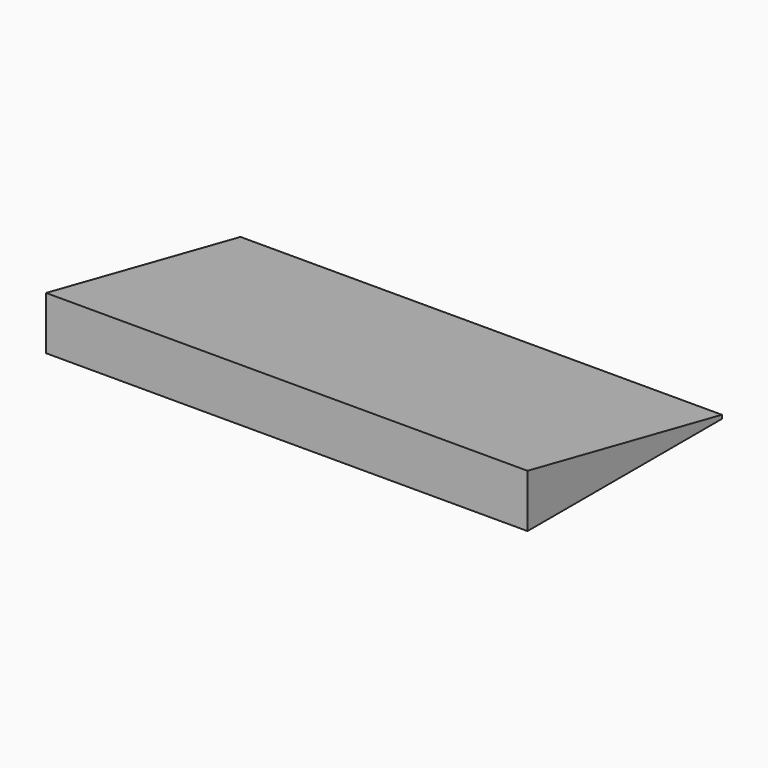
from build123d import *

# Parameters (mm, degrees)
F0_W     = 107
F0_H     = 54
F1_DEPTH = 11.8
F2_SIZE2 = 10.986414
F2_SIZE  = 53.99999


# Not quite as in the source:
# - a fillet or chamfer is up to 0.001 mm smaller than in the source, because OpenCascade refuses the exact size


with BuildPart() as f1:
    # F0 (on Top) → F1 (new body)
    with BuildSketch(Plane.XY):
        with Locations((53.5, -27)):
            Rectangle(F0_W, F0_H)
    extrude(amount=F1_DEPTH)

    # F2 (size 54 and 10.9864241689 in the source; OpenCascade refuses exactly that, so slightly less here)
    f2_edges = [f1.edges().sort_by_distance(p)[0] for p in [
        (53.5, 0, 11.8),
    ]]
    f2_side = f1.faces().sort_by_distance((53.5, -27, 11.8))[0]
    chamfer(f2_edges, length=F2_SIZE, length2=F2_SIZE2, reference=f2_side)


solid = f1.part
